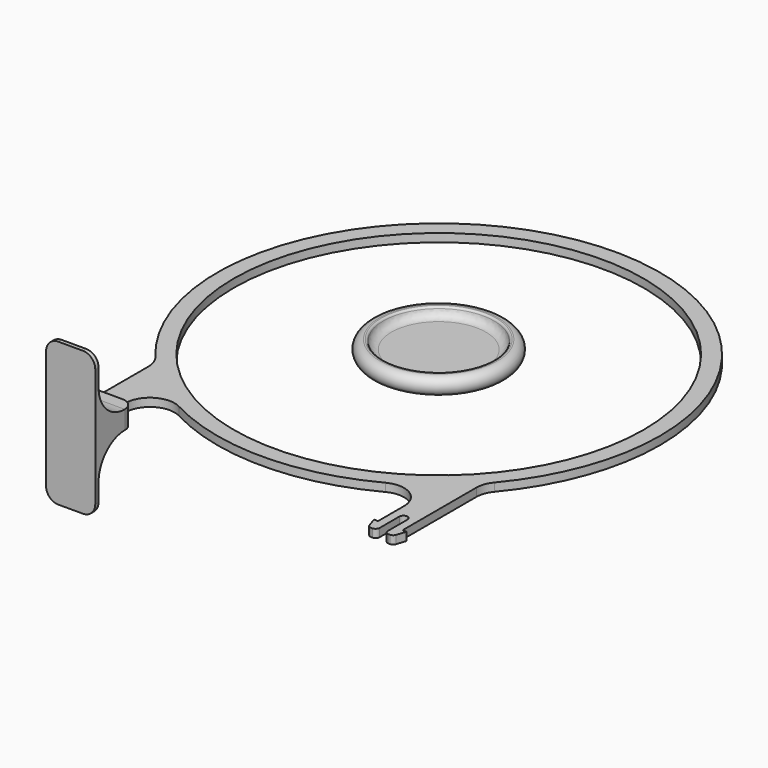
from build123d import *

# Parameters (mm, degrees)
F2_R         = 0.5
F3_R         = 2
F4_R         = 50
F5_DEPTH     = 1
F6_R         = 6
F7_W         = 12
F7_H         = 12
F8_DEPTH     = 2.25
F9_W         = 6.3
F9_H         = 2.3
F9_W_2       = 6
F9_H_2       = 2
F10_DEPTH    = 7
F11_START    = -7
F9_W_3       = 0.8
F11_DEPTH    = 4
F12_W        = 12
F12_H        = 1
F13_DEPTH    = 17.5
F14_R        = 8
F15_T1_DEPTH = 19.5
F15_T3_DEPTH = 16


# Not quite as in the source:
# - a fillet or chamfer that OpenCascade refuses, or shapes differently, is made with other operations: its cross-section is extruded or revolved along the edge and cut away or added


with BuildPart() as f1:
    # F0 (on Front) → F1 (revolve)
    with BuildSketch(Plane.XZ):
        with BuildLine():
            Line((-14.35, 0), (0, 0))
            Line((0, 0), (0, 2))
            Line((0, 2), (-13.5, 2))
            Line((-13.5, 2), (-13.5, 4.2))
            Line((-13.5, 4.2), (-14.35, 4.2))
            ThreePointArc((-14.35, 4.2), (-16.45, 2.1), (-14.35, 0))
        make_face()
    revolve(axis=Axis((0, 0, 1), (0, 0, -1)))

    # F2
    f2_edges = [f1.edges().sort_by_distance(p)[0] for p in [
        (13.5, 0, 4.2),
    ]]
    fillet(f2_edges, radius=F2_R)

    # F3
    f3_edges = [f1.edges().sort_by_distance(p)[0] for p in [
        (13.5, 0, 2),
    ]]
    fillet(f3_edges, radius=F3_R)


with BuildPart() as f5:
    # F4 (on Top) → F5 (new body, symmetric)
    with BuildSketch(Plane.XY):
        with BuildLine():
            ThreePointArc((40, -36.2767142944), (50.3785668712, -19.4422220952), (54, 0))
            ThreePointArc((54, 0), (-19.4422220952, 50.3785668712), (-40, -36.2767142944))
            ThreePointArc((-40, -36.2767142944), (-37.1086677383, -39.2294121635), (-34, -41.9523539268))
            ThreePointArc((-34, -41.9523539268), (0, -54), (34, -41.9523539268))
            ThreePointArc((34, -41.9523539268), (37.1086677383, -39.2294121635), (40, -36.2767142944))
        make_face()
        Circle(F4_R, mode=Mode.SUBTRACT)
        with BuildLine():
            ThreePointArc((-34, -41.9523539268), (-37.1086677383, -39.2294121635), (-40, -36.2767142944))
            Line((-40, -36.2767142944), (-40, -61))
            Line((-40, -61), (-41, -61))
            Line((-41, -61), (-40.227924078, -63.316227766))
            ThreePointArc((-40.227924078, -63.316227766), (-39.8639510646, -63.8112421852), (-39.2792407799, -64))
            Line((-39.2792407799, -64), (-39, -64))
            ThreePointArc((-39, -64), (-38.2928932188, -63.7071067812), (-38, -63))
            Line((-38, -63), (-38, -57))
            ThreePointArc((-38, -57), (-37.7071067812, -56.2928932188), (-37, -56))
            ThreePointArc((-37, -56), (-36.2928932188, -56.2928932188), (-36, -57))
            Line((-36, -57), (-36, -63))
            ThreePointArc((-36, -63), (-35.7071067812, -63.7071067812), (-35, -64))
            Line((-35, -64), (-34.7207592201, -64))
            ThreePointArc((-34.7207592201, -64), (-34.1360489354, -63.8112421852), (-33.772075922, -63.316227766))
            Line((-33.772075922, -63.316227766), (-33, -61))
            Line((-33, -61), (-34, -61))
            Line((-34, -61), (-34, -41.9523539268))
        make_face()
        with BuildLine():
            Line((40, -61), (40, -36.2767142944))
            ThreePointArc((40, -36.2767142944), (37.1086677383, -39.2294121635), (34, -41.9523539268))
            Line((34, -41.9523539268), (34, -61))
            Line((34, -61), (33, -61))
            Line((33, -61), (33.772075922, -63.316227766))
            ThreePointArc((33.772075922, -63.316227766), (34.1360489354, -63.8112421852), (34.7207592201, -64))
            Line((34.7207592201, -64), (35, -64))
            ThreePointArc((35, -64), (35.7071067812, -63.7071067812), (36, -63))
            Line((36, -63), (36, -57))
            ThreePointArc((36, -57), (36.2928932188, -56.2928932188), (37, -56))
            ThreePointArc((37, -56), (37.7071067812, -56.2928932188), (38, -57))
            Line((38, -57), (38, -63))
            ThreePointArc((38, -63), (38.2928932188, -63.7071067812), (39, -64))
            Line((39, -64), (39.2792407799, -64))
            ThreePointArc((39.2792407799, -64), (39.8639510646, -63.8112421852), (40.227924078, -63.316227766))
            Line((40.227924078, -63.316227766), (41, -61))
            Line((41, -61), (40, -61))
        make_face()
    extrude(amount=F5_DEPTH, both=True)

    # F6
    f6_edges = [f5.edges().sort_by_distance(p)[0] for p in [
        (-34, -41.952354, 0),
        (-40, -36.276714, 0),
        (40, -36.276714, 0),
        (34, -41.952354, 0),
    ]]
    fillet(f6_edges, radius=F6_R)


with BuildPart() as f8:
    # F7 (on Top) → F8 (new body, symmetric)
    with BuildSketch(Plane.XY):
        with Locations((-37, -60)):
            Rectangle(F7_W, F7_H)
    extrude(amount=F8_DEPTH, both=True)

    # F9 (on face) → F10 (cut)
    with BuildSketch(Plane(origin=(0, -54, 0), x_dir=(-1, 0, 0), z_dir=(0, 1, 0))):
        with Locations((37, 0)):
            Rectangle(F9_W, F9_H)
        with Locations((37, 0)):
            Rectangle(F9_W_2, F9_H_2, mode=Mode.SUBTRACT)
        with Locations((37, 0)):
            Rectangle(F9_W_2, F9_H_2)
    extrude(amount=-F10_DEPTH, mode=Mode.SUBTRACT)

    # F9 (on face) → F11 (cut)
    with BuildSketch(Plane(origin=(0, -54, 0), x_dir=(-1, 0, 0), z_dir=(0, 1, 0)).offset(F11_START)):
        with Locations((40.55, 0)):
            Rectangle(F9_W_3, F9_H)
        with Locations((37, 0)):
            Rectangle(F9_W, F9_H)
        with Locations((37, 0)):
            Rectangle(F9_W_2, F9_H_2, mode=Mode.SUBTRACT)
        with Locations((37, 0)):
            Rectangle(F9_W_2, F9_H_2)
        with Locations((33.45, 0)):
            Rectangle(F9_W_3, F9_H)
    extrude(amount=-F11_DEPTH, mode=Mode.SUBTRACT)

    # F12 (on Top) → F13 (join, symmetric)
    with BuildSketch(Plane.XY):
        with Locations((-37, -65.5)):
            Rectangle(F12_W, F12_H)
    extrude(amount=F13_DEPTH, both=True)

    # F14
    f14_edges = [f8.edges().sort_by_distance(p)[0] for p in [
        (-37, -65, -2.25),
        (-37, -65, 2.25),
    ]]
    fillet(f14_edges, radius=F14_R)

    # F15: fillet of radius 3 on 6 edges, made by hand

    # F15_s2 → F15_t1 (cut)
    with BuildSketch(Plane.XY.offset(-9.75)):
        with BuildLine():
            ThreePointArc((-34, -54), (-31.8786796564, -54.8786796564), (-31, -57))
            Line((-31, -57), (-31, -54))
            Line((-31, -54), (-34, -54))
        make_face()
        with BuildLine():
            ThreePointArc((-43, -57), (-42.1213203436, -54.8786796564), (-40, -54))
            Line((-40, -54), (-43, -54))
            Line((-43, -54), (-43, -57))
        make_face()
    extrude(amount=F15_T1_DEPTH, mode=Mode.SUBTRACT)

    # F15_s4 → F15_t3 (cut)
    with BuildSketch(Plane.XZ.offset(57.5)):
        with BuildLine():
            ThreePointArc((-43, 14.5), (-42.1213203436, 16.6213203436), (-40, 17.5))
            Line((-40, 17.5), (-43, 17.5))
            Line((-43, 17.5), (-43, 14.5))
        make_face()
        with BuildLine():
            ThreePointArc((-34, 17.5), (-31.8786796564, 16.6213203436), (-31, 14.5))
            Line((-31, 14.5), (-31, 17.5))
            Line((-31, 17.5), (-34, 17.5))
        make_face()
        with BuildLine():
            ThreePointArc((-43, -14.5), (-42.1213203436, -16.6213203436), (-40, -17.5))
            Line((-40, -17.5), (-43, -17.5))
            Line((-43, -17.5), (-43, -14.5))
        make_face()
        with BuildLine():
            ThreePointArc((-34, -17.5), (-31.8786796564, -16.6213203436), (-31, -14.5))
            Line((-31, -14.5), (-31, -17.5))
            Line((-31, -17.5), (-34, -17.5))
        make_face()
    extrude(amount=F15_T3_DEPTH, mode=Mode.SUBTRACT)


solid = Compound([f1.part, f5.part, f8.part])
